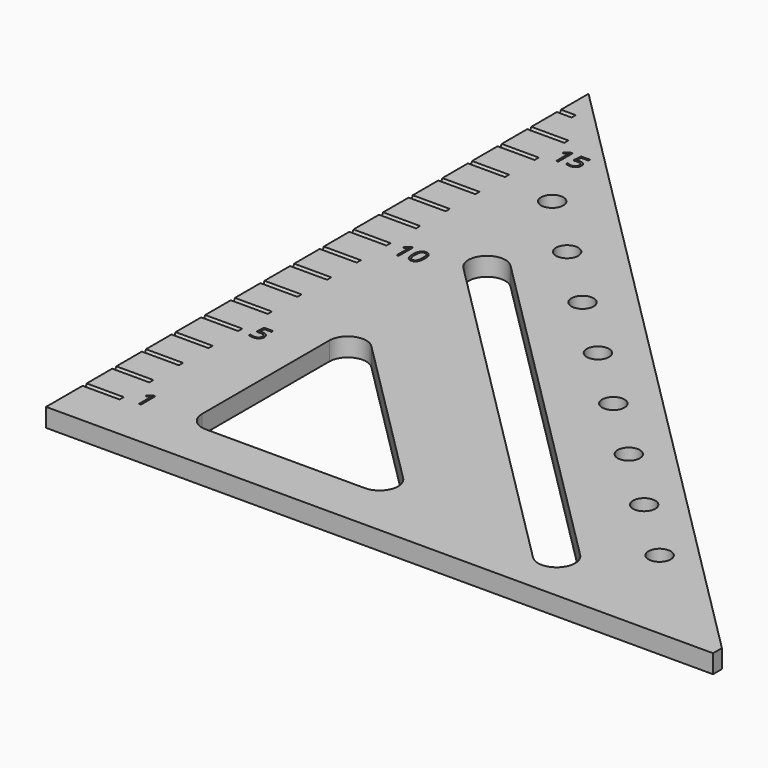
from build123d import *

# Parameters (mm, degrees)
F0_W         = 179.9989728027
F0_H         = 3
F1_DEPTH     = 2.5
F4_DEPTH     = 10
F5_DEPTH     = 4
F7_R         = 3
F8_DEPTH     = 10
F7_TEXT_SIZE = 6.8211552141
F9_DEPTH     = 1
F10_DEPTH    = 12.5
F11_DEPTH    = 5.001


# Not quite as in the source:
# - Text() gives the source's letters only with a copy of the font that has no kerning and outlines rounded to 1/6400 em; it was checked with that copy


with BuildPart() as f1:
    # F0 (on Top) → F1 (new body, symmetric)
    with BuildSketch(Plane.XY):
        Polygon((-55.4096413546, 107.5159661705), (-55.4096413546, -72.4840338295), (124.5893314481, -72.4840338295), (124.5903586454, -72.4840338295), (86.5518828724, -34.4455580566), (58.7057859642, -6.5994611483), (34.5903586454, 17.5159661705), (10.4749313266, 41.6313934893), (-17.3711655817, 69.4774903975), align=None)
        with BuildLine():
            Line((-27.7254325097, -57.4840338295), (-27.7254325097, -14.5551016414))
            ThreePointArc((-27.7254325097, -14.5551016414), (-24.6388496715, -9.9357039788), (-19.1898986038, -11.0195677355))
            Line((-19.1898986038, -11.0195677355), (23.7390335844, -53.9484999236))
            ThreePointArc((23.7390335844, -53.9484999236), (24.822897341, -59.3974509913), (20.2034996784, -62.4840338295))
            Line((20.2034996784, -62.4840338295), (-22.7254325097, -62.4840338295))
            ThreePointArc((-22.7254325097, -62.4840338295), (-26.2609664156, -61.0195677355), (-27.7254325097, -57.4840338295))
        make_face(mode=Mode.SUBTRACT)
        with BuildLine():
            ThreePointArc((-26.3397537637, 28.9486038965), (-26.3397537637, 36.0196717083), (-19.2686859518, 36.0196717083))
            Line((-19.2686859518, 36.0196717083), (74.776515946, -58.0255301895))
            ThreePointArc((74.776515946, -58.0255301895), (74.776515946, -65.0965980013), (67.7054481341, -65.0965980013))
            Line((67.7054481341, -65.0965980013), (-26.3397537637, 28.9486038965))
        make_face(mode=Mode.SUBTRACT)
        with Locations((34.5898450467, -73.9840338295)):
            Rectangle(F0_W, F0_H)
    extrude(amount=F1_DEPTH, both=True)

    # F3 (on offset) → F4 (cut)
    with BuildSketch(Plane(origin=(-55.4096413546, 0, 0), x_dir=(0, -1, 0), z_dir=(-1, 0, 0))):
        Polygon((63.1840338295, 2.5128277827), (62.4840338295, 2.5128277827), (61.7840338295, 2.5128277827), (62.4840338295, 1.1861778665), align=None)
        Polygon((52.4840338295, 2.5128277827), (51.7840338295, 2.5128277827), (52.4840338295, 1.1861778665), (53.1840338295, 2.5128277827), align=None)
        Polygon((42.4840338295, 2.5128277827), (41.7840338295, 2.5128277827), (42.4840338295, 1.1861778665), (43.1840338295, 2.5128277827), align=None)
        Polygon((32.4840338295, 2.5128277827), (31.7840338295, 2.5128277827), (32.4840338295, 1.1861778665), (33.1840338295, 2.5128277827), align=None)
        Polygon((22.4840338295, 2.5128277827), (21.7840338295, 2.5128277827), (22.4840338295, 1.1861778665), (23.1840338295, 2.5128277827), align=None)
        Polygon((12.4840338295, 2.5128277827), (11.7840338295, 2.5128277827), (12.4840338295, 1.1861778665), (13.1840338295, 2.5128277827), align=None)
        Polygon((2.4840338295, 2.5128277827), (1.7840338295, 2.5128277827), (2.4840338295, 1.1861778665), (3.1840338295, 2.5128277827), align=None)
        Polygon((-7.5159661705, 2.5128277827), (-8.2159661705, 2.5128277827), (-7.5159661705, 1.1861778665), (-6.8159661705, 2.5128277827), align=None)
        Polygon((-17.5159661705, 2.5128277827), (-18.2159661705, 2.5128277827), (-17.5159661705, 1.1861778665), (-16.8159661705, 2.5128277827), align=None)
        Polygon((-27.5159661705, 2.5128277827), (-28.2159661705, 2.5128277827), (-27.5159661705, 1.1861778665), (-26.8159661705, 2.5128277827), align=None)
        Polygon((-37.5159661705, 2.5128277827), (-38.2159661705, 2.5128277827), (-37.5159661705, 1.1861778665), (-36.8159661705, 2.5128277827), align=None)
        Polygon((-47.5159661705, 2.5128277827), (-48.2159661705, 2.5128277827), (-47.5159661705, 1.1861778665), (-46.8159661705, 2.5128277827), align=None)
        Polygon((-57.5159661705, 2.5128277827), (-58.2159661705, 2.5128277827), (-57.5159661705, 1.1861778665), (-56.8159661705, 2.5128277827), align=None)
        Polygon((-67.5159661705, 2.5128277827), (-68.2159661705, 2.5128277827), (-67.5159661705, 1.1861778665), (-66.8159661705, 2.5128277827), align=None)
        Polygon((-77.5159661705, 2.5128277827), (-78.2159661705, 2.5128277827), (-77.5159661705, 1.1861778665), (-76.8159661705, 2.5128277827), align=None)
        Polygon((-87.5159661705, 2.5128277827), (-88.2159661705, 2.5128277827), (-87.5159661705, 1.1861778665), (-86.8159661705, 2.5128277827), align=None)
    extrude(amount=-F4_DEPTH, mode=Mode.SUBTRACT)

    # F3 (on offset) → F5 (cut)
    with BuildSketch(Plane(origin=(-55.4096413546, 0, 0), x_dir=(0, -1, 0), z_dir=(-1, 0, 0))):
        Polygon((-97.5159661705, 2.5128277827), (-98.2159661705, 2.5128277827), (-97.5159661705, 1.1861778665), (-96.8159661705, 2.5128277827), align=None)
    extrude(amount=-F5_DEPTH, mode=Mode.SUBTRACT)

    # F7 (on offset) → F8 (cut)
    with BuildSketch(Plane.XY.offset(2.5)):
        with Locations((-30.7070528007, 64.3810529124)):
            Circle(F7_R)
    extrude(amount=-F8_DEPTH, mode=Mode.SUBTRACT)

    # F7 (on offset) → F9 (cut)
    with BuildSketch(Plane.XY.offset(2.5)):
        with Locations((-30.7070528007, 64.3810529124)):
            Circle(F7_R)
        with Locations((-13.8854532777, 48.3810529124)):
            Circle(F7_R)
        with Locations((3.0747424225, 32.3810529124)):
            Circle(F7_R)
        with Locations((20.0349381227, 16.3810529124)):
            Circle(F7_R)
        with Locations((36.995133823, 0.3810529124)):
            Circle(F7_R)
        with Locations((53.9553295232, -15.6189470876)):
            Circle(F7_R)
        with Locations((70.9155252234, -31.6189470876)):
            Circle(F7_R)
        with Locations((87.8757209236, -47.6189470876)):
            Circle(F7_R)
        with Locations((-42.8156469105, -62.2108423145)):
            Text('1', F7_TEXT_SIZE, font='Open Sans', text_align=(TextAlign.LEFT, TextAlign.BOTTOM))
        with Locations((-42.8124668382, 24.7411911504)):
            Text('10', F7_TEXT_SIZE, font='Open Sans', text_align=(TextAlign.LEFT, TextAlign.BOTTOM))
        with Locations((-42.8338362052, -23.4495665993)):
            Text('5', F7_TEXT_SIZE, font='Open Sans', text_align=(TextAlign.LEFT, TextAlign.BOTTOM))
        with Locations((-43.4145964551, 79.3297764066)):
            Text('15', F7_TEXT_SIZE, font='Open Sans', text_align=(TextAlign.LEFT, TextAlign.BOTTOM))
    extrude(amount=-F9_DEPTH, mode=Mode.SUBTRACT)

    # F7 (on offset) → F10 (cut, symmetric)
    with BuildSketch(Plane.XY.offset(2.5)):
        with Locations((-30.7070528007, 64.3810529124)):
            Circle(F7_R)
    extrude(amount=F10_DEPTH, both=True, mode=Mode.SUBTRACT)

    # F7 (on offset) → F11 (cut, through all)
    with BuildSketch(Plane.XY.offset(2.5)):
        with Locations((-30.7070528007, 64.3810529124)):
            Circle(F7_R)
        with Locations((-13.8854532777, 48.3810529124)):
            Circle(F7_R)
        with Locations((3.0747424225, 32.3810529124)):
            Circle(F7_R)
        with Locations((20.0349381227, 16.3810529124)):
            Circle(F7_R)
        with Locations((36.995133823, 0.3810529124)):
            Circle(F7_R)
        with Locations((53.9553295232, -15.6189470876)):
            Circle(F7_R)
        with Locations((70.9155252234, -31.6189470876)):
            Circle(F7_R)
        with Locations((87.8757209236, -47.6189470876)):
            Circle(F7_R)
    extrude(amount=-F11_DEPTH, mode=Mode.SUBTRACT)


solid = f1.part
